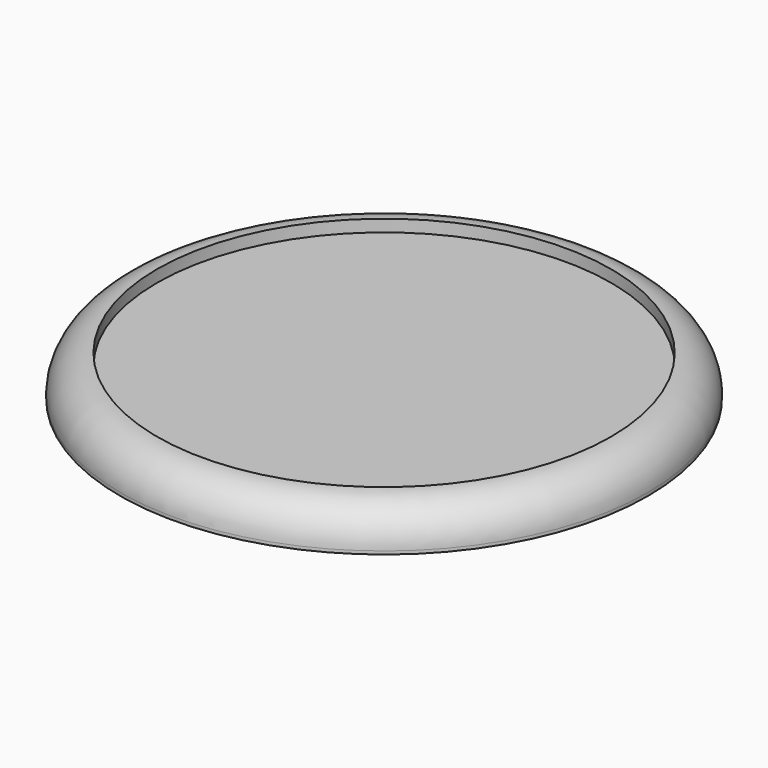
from build123d import *

# Parameters (mm, degrees)
F0_R     = 25
F0_R_2   = 21.5
F1_DEPTH = 3.8
F2_DEPTH = 2.66
F3_R     = 3.49999
F4_R     = 1.6
F5_DEPTH = 1.9
F6_DEPTH = 1.66
F6_TAPER = 25


# Not quite as in the source:
# - a fillet or chamfer is up to 0.001 mm smaller than in the source, because OpenCascade refuses the exact size


with BuildPart() as f1:
    # F0 (on Top) → F1 (new body)
    with BuildSketch(Plane.XY):
        Circle(F0_R)
        Circle(F0_R_2, mode=Mode.SUBTRACT)
    extrude(amount=F1_DEPTH)

    # F0 (on Top) → F2 (join, through all)
    with BuildSketch(Plane.XY):
        Circle(F0_R_2)
    extrude(amount=F2_DEPTH)

    # F3 (radius 3.5 in the source; OpenCascade refuses exactly that, so slightly less here)
    f3_edges = [f1.edges().sort_by_distance(p)[0] for p in [
        (-25, 0, 3.8),
    ]]
    fillet(f3_edges, radius=F3_R)

    # F4 (on face) → F5 (cut)
    with BuildSketch(Plane.XY):
        Circle(F4_R)
    extrude(amount=F5_DEPTH, mode=Mode.SUBTRACT)

    # F4 (on face) → F6 (cut, through all)
    with BuildSketch(Plane.XY):
        with BuildLine():
            Line((-1, -21.4767315949), (-1, -3.4583232932))
            ThreePointArc((-1, -3.4583232932), (-2.1160269083, -2.9124611797), (-2.980043909, -2.0197371859))
            Line((-2.980043909, -2.0197371859), (-20.1165685377, -7.5877315628))
            ThreePointArc((-20.1165685377, -7.5877315628), (-12.6373829243, -17.3938653791), (-1, -21.4767315949))
        make_face()
        with BuildLine():
            Line((-1, -21.9772609758), (-1, -21.4767315949))
            ThreePointArc((-1, -21.4767315949), (-12.6373829243, -17.3938653791), (-20.1165685377, -7.5877315628))
            Line((-20.1165685377, -7.5877315628), (-20.592600267, -7.7424036476))
            ThreePointArc((-20.592600267, -7.7424036476), (-12.9312755504, -17.7983738762), (-1, -21.9772609758))
        make_face()
        with BuildLine():
            Line((20.1165685377, -7.5877315628), (2.980043909, -2.0197371859))
            ThreePointArc((2.980043909, -2.0197371859), (2.1160269083, -2.9124611797), (1, -3.4583232932))
            Line((1, -3.4583232932), (1, -21.4767315949))
            ThreePointArc((1, -21.4767315949), (12.6373829243, -17.3938653791), (20.1165685377, -7.5877315628))
        make_face()
        with BuildLine():
            Line((20.592600267, -7.7424036476), (20.1165685377, -7.5877315628))
            ThreePointArc((20.1165685377, -7.5877315628), (12.6373829243, -17.3938653791), (1, -21.4767315949))
            Line((1, -21.4767315949), (1, -21.9772609758))
            ThreePointArc((1, -21.9772609758), (12.9312755504, -17.7983738762), (20.592600267, -7.7424036476))
        make_face()
        with BuildLine():
            ThreePointArc((2.8417684238, 2.2100570639), (3.4051700637, 1.1682537555), (3.6, 0))
            ThreePointArc((3.6, 0), (3.5995194424, -0.0588199284), (3.5980778978, -0.1176241533))
            Line((3.5980778978, -0.1176241533), (20.7346025264, -5.6856185302))
            ThreePointArc((20.7346025264, -5.6856185302), (21.307791466, -2.8684530397), (21.5, 0))
            ThreePointArc((21.5, 0), (19.3785131848, 9.3125306307), (13.4327230933, 16.7872555916))
            Line((13.4327230933, 16.7872555916), (2.8417684238, 2.2100570639))
        make_face()
        with BuildLine():
            Line((13.7269268818, 17.192192367), (13.4327230933, 16.7872555916))
            ThreePointArc((13.4327230933, 16.7872555916), (19.3785131848, 9.3125306307), (21.5, 0))
            ThreePointArc((21.5, 0), (21.307791466, -2.8684530397), (20.7346025264, -5.6856185302))
            Line((20.7346025264, -5.6856185302), (21.2106342558, -5.8402906151))
            ThreePointArc((21.2106342558, -5.8402906151), (21.8017654518, -2.9466969961), (22, 0))
            ThreePointArc((22, 0), (19.8241316506, 9.5395914116), (13.7269268818, 17.192192367))
        make_face()
        with BuildLine():
            ThreePointArc((-1.223734435, 3.3856275685), (0, 3.6), (1.223734435, 3.3856275685))
            Line((1.223734435, 3.3856275685), (11.8146891046, 17.9628260962))
            ThreePointArc((11.8146891046, 17.9628260962), (0, 21.5), (-11.8146891046, 17.9628260962))
            Line((-11.8146891046, 17.9628260962), (-1.223734435, 3.3856275685))
        make_face()
        with BuildLine():
            ThreePointArc((-11.8146891046, 17.9628260962), (0, 21.5), (11.8146891046, 17.9628260962))
            Line((11.8146891046, 17.9628260962), (12.108892893, 18.3677628716))
            ThreePointArc((12.108892893, 18.3677628716), (0, 22), (-12.108892893, 18.3677628716))
            Line((-12.108892893, 18.3677628716), (-11.8146891046, 17.9628260962))
        make_face()
        with BuildLine():
            ThreePointArc((-3.5980778978, -0.1176241533), (-3.4238034587, 1.1124611797), (-2.8417684238, 2.2100570639))
            Line((-2.8417684238, 2.2100570639), (-13.4327230933, 16.7872555916))
            ThreePointArc((-13.4327230933, 16.7872555916), (-20.4477151003, 6.6438653791), (-20.7346025264, -5.6856185302))
            Line((-20.7346025264, -5.6856185302), (-3.5980778978, -0.1176241533))
        make_face()
        with BuildLine():
            ThreePointArc((-20.7346025264, -5.6856185302), (-20.4477151003, 6.6438653791), (-13.4327230933, 16.7872555916))
            Line((-13.4327230933, 16.7872555916), (-13.7269268818, 17.192192367))
            ThreePointArc((-13.7269268818, 17.192192367), (-20.9232433585, 6.7983738762), (-21.2106342558, -5.8402906151))
            Line((-21.2106342558, -5.8402906151), (-20.7346025264, -5.6856185302))
        make_face()
    extrude(amount=F6_DEPTH, taper=F6_TAPER, mode=Mode.SUBTRACT)


solid = f1.part
